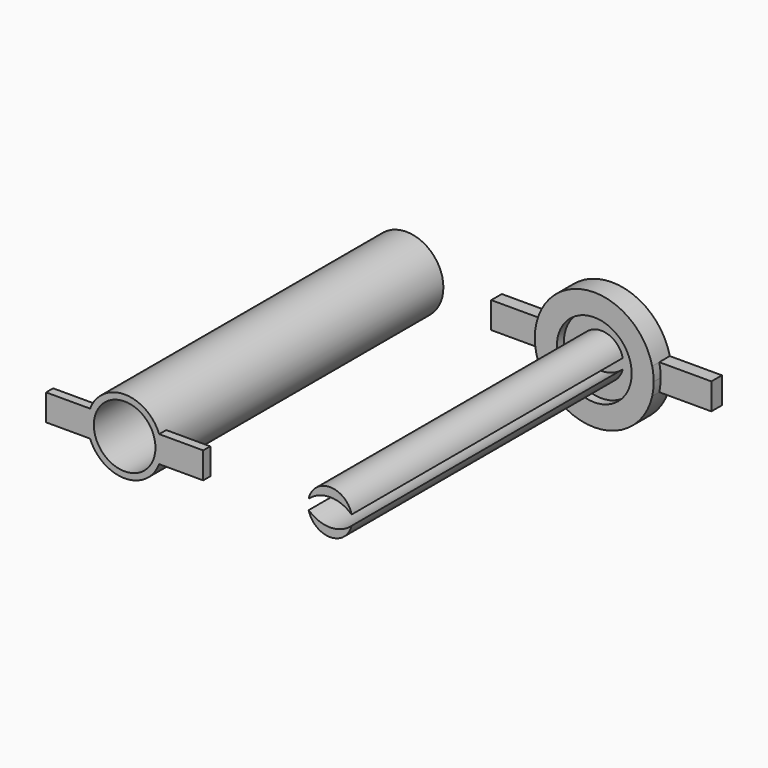
from build123d import *

# Parameters (mm, degrees)
F0_R     = 15.875
F1_DEPTH = 3.81
F2_R     = 10.795
F3_DEPTH = 2.54
F4_R     = 10.668
F4_R_2   = 8.89
F5_DEPTH = 101.6
F7_DEPTH = 101.6
F9_DEPTH = 2.54


# Not quite as in the source:
# - a feature names something its author has since deleted; it is built from what else it names


with BuildPart() as f1:
    # F0 (on Front) → F1 (new body)
    with BuildSketch(Plane.XZ):
        with BuildLine():
            Line((34.2841744423, 3.81), (34.2841744423, 0))
            Line((34.2841744423, 0), (34.2841744423, -3.81))
            Line((34.2841744423, -3.81), (49.3178672843, -3.81))
            ThreePointArc((49.3178672843, -3.81), (48.8891744423, 0), (49.3178672843, 3.81))
            Line((49.3178672843, 3.81), (34.2841744423, 3.81))
        make_face()
        with BuildLine():
            Line((97.7841744423, 3.81), (82.7504816003, 3.81))
            ThreePointArc((82.7504816003, 3.81), (83.0716641521, 1.9170209671), (83.1791744423, 0))
            ThreePointArc((83.1791744423, 0), (83.0716641521, -1.9170209671), (82.7504816003, -3.81))
            Line((82.7504816003, -3.81), (97.7841744423, -3.81))
            Line((97.7841744423, -3.81), (97.7841744423, 0))
            Line((97.7841744423, 0), (97.7841744423, 3.81))
        make_face()
        with BuildLine():
            ThreePointArc((82.7504816003, 3.81), (66.0341744423, 17.145), (49.3178672843, 3.81))
            ThreePointArc((49.3178672843, 3.81), (48.8891744423, 0), (49.3178672843, -3.81))
            ThreePointArc((49.3178672843, -3.81), (66.0341744423, -17.145), (82.7504816003, -3.81))
            ThreePointArc((82.7504816003, -3.81), (83.0716641521, -1.9170209671), (83.1791744423, 0))
            ThreePointArc((83.1791744423, 0), (83.0716641521, 1.9170209671), (82.7504816003, 3.81))
        make_face()
        with Locations((66.0341744423, 0)):
            Circle(F0_R, mode=Mode.SUBTRACT)
        with Locations((66.0341744423, 0)):
            Circle(F0_R)
    extrude(amount=F1_DEPTH)

    # F2 (on face) → F3 (join)
    with BuildSketch(Plane.XZ.offset(3.81)):
        with BuildLine():
            ThreePointArc((82.7504816003, 3.81), (66.0341744423, 17.145), (49.3178672843, 3.81))
            ThreePointArc((49.3178672843, 3.81), (48.8891744423, 0), (49.3178672843, -3.81))
            ThreePointArc((49.3178672843, -3.81), (66.0341744423, -17.145), (82.7504816003, -3.81))
            ThreePointArc((82.7504816003, -3.81), (83.0716641521, -1.9170209671), (83.1791744423, 0))
            ThreePointArc((83.1791744423, 0), (83.0716641521, 1.9170209671), (82.7504816003, 3.81))
        make_face()
        with Locations((66.0341744423, 0)):
            Circle(F2_R, mode=Mode.SUBTRACT)
    extrude(amount=F3_DEPTH)

    # F6 (on Front) → F7 (join)
    with BuildSketch(Plane.XZ):
        with BuildLine():
            ThreePointArc((66.0341744423, 3.8478664845), (69.3580825337, 3.2233188982), (72.2285986286, 1.4348664845))
            ThreePointArc((72.2285986286, 1.4348664845), (66.0341744423, 6.3878664845), (59.839750256, 1.4348664845))
            ThreePointArc((59.839750256, 1.4348664845), (62.7102663509, 3.2233188982), (66.0341744423, 3.8478664845))
        make_face()
        with BuildLine():
            ThreePointArc((59.8622690304, -1.4554799544), (66.0341744423, -6.3121335155), (72.2060798542, -1.4554799544))
            ThreePointArc((72.2060798542, -1.4554799544), (66.0341744423, -3.8478664845), (59.8622690304, -1.4554799544))
        make_face()
    extrude(amount=F7_DEPTH)


with BuildPart() as f5:
    # F4 (on Front) → F5 (new body)
    with BuildSketch(Plane.XZ):
        with Locations((6.7617367022, 0)):
            Circle(F4_R)
        with Locations((6.7617367022, 0)):
            Circle(F4_R_2, mode=Mode.SUBTRACT)
    extrude(amount=F5_DEPTH)

    # F8 (on face) → F9 (join)
    with BuildSketch(Plane.XZ.offset(101.6)):
        with BuildLine():
            ThreePointArc((-3.2027062828, -3.81), (-3.9062632978, 0), (-3.2027062828, 3.81))
            Line((-3.2027062828, 3.81), (-15.9027062828, 3.81))
            Line((-15.9027062828, 3.81), (-15.9027062828, -3.81))
            Line((-15.9027062828, -3.81), (-3.2027062828, -3.81))
        make_face()
        with BuildLine():
            Line((29.4261796871, 3.81), (16.7261796871, 3.81))
            ThreePointArc((16.7261796871, 3.81), (17.2523730452, 1.9372075569), (17.4297367022, 0))
            ThreePointArc((17.4297367022, 0), (17.2523730452, -1.9372075569), (16.7261796871, -3.81))
            Line((16.7261796871, -3.81), (29.4261796871, -3.81))
            Line((29.4261796871, -3.81), (29.4261796871, 3.81))
        make_face()
    extrude(amount=-F9_DEPTH)


solid = Compound([f1.part, f5.part])
